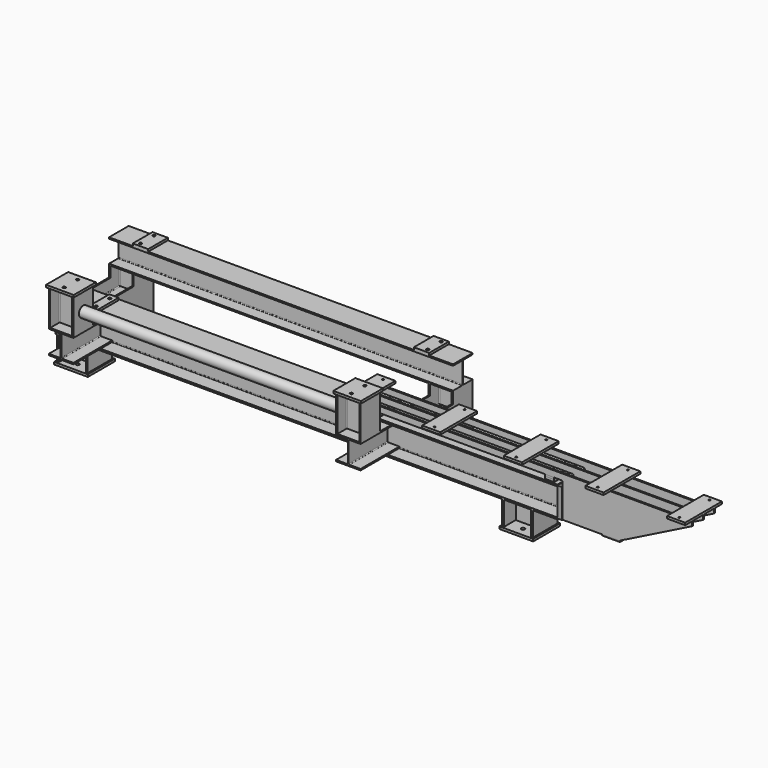
from build123d import *

# Parameters (mm, degrees)
F0_W       = 228.6
F0_H       = 228.6
F0_R       = 14.2875
F1_DEPTH   = 19.05
F0_W_2     = 279.4
F0_H_2     = 279.4
F3_DEPTH   = 504.952
F5_DEPTH   = 2844.8
F6_W       = 127
F6_H       = 203.2
F6_R       = 11.1125
F7_DEPTH   = 19.05
F9_DEPTH   = 482.6
F12_DEPTH  = 4152.9
F14_DEPTH  = 198.374
F15_W      = 76.2
F15_H      = 228.6
F15_R      = 11.1125
F16_DEPTH  = 19.05
F18_DEPTH  = 401.574
F20_DEPTH  = 292.1
F21_W      = 228.6
F21_H      = 228.6
F21_R      = 11.1125
F22_DEPTH  = 19.05
F23_R      = 44.45
F23_R_2    = 38.9636
F24_DEPTH  = 2171.7
F25_W      = 76.2
F25_H      = 228.6
F25_R      = 11.1125
F26_DEPTH  = 19
F28_W      = 150
F28_H      = 380
F28_R      = 7.25
F29_DEPTH  = 19
F31_W      = 254
F31_H      = 239.776
F31_R      = 10
F32_DEPTH  = 19
F33_W      = 254
F33_H      = 239.776
F33_R      = 10
F34_DEPTH  = 19
F36_DEPTH  = 6.25
F38_DEPTH  = 6.25
F39_SIZE2  = 600
F39_SIZE   = 300
F41_SIZE   = 40
F41_2_SIZE = 40
F43_W      = 150
F43_H      = 228.6
F44_DEPTH  = 12.5


with BuildPart() as f1:
    # F0 (on Top) → F1 (new body)
    with BuildSketch(Plane.XY):
        with Locations((-1320.8, 241.3)):
            Rectangle(F0_W, F0_H)
        with Locations((-1320.8, 171.45)):
            Circle(F0_R, mode=Mode.SUBTRACT)
        with Locations((-1320.8, 311.15)):
            Circle(F0_R, mode=Mode.SUBTRACT)
    extrude(amount=F1_DEPTH)

    # F2 (on face) → F3 (join)
    with BuildSketch(Plane.XY.offset(19.05)):
        with BuildLine():
            Line((-1411.351, 342.9), (-1422.4, 342.9))
            Line((-1422.4, 342.9), (-1422.4, 139.7))
            Line((-1422.4, 139.7), (-1411.351, 139.7))
            Line((-1411.351, 139.7), (-1411.351, 231.3305))
            ThreePointArc((-1411.351, 231.3305), (-1409.4911280605, 235.8206280605), (-1405.001, 237.6805))
            Line((-1405.001, 237.6805), (-1320.8, 237.6805))
            Line((-1320.8, 237.6805), (-1236.599, 237.6805))
            ThreePointArc((-1236.599, 237.6805), (-1232.1088719395, 235.8206280605), (-1230.249, 231.3305))
            Line((-1230.249, 231.3305), (-1230.249, 139.7))
            Line((-1230.249, 139.7), (-1219.2, 139.7))
            Line((-1219.2, 139.7), (-1219.2, 342.9))
            Line((-1219.2, 342.9), (-1230.249, 342.9))
            Line((-1230.249, 342.9), (-1230.249, 251.2695))
            ThreePointArc((-1230.249, 251.2695), (-1232.1088719395, 246.7793719395), (-1236.599, 244.9195))
            Line((-1236.599, 244.9195), (-1320.8, 244.9195))
            Line((-1320.8, 244.9195), (-1405.001, 244.9195))
            ThreePointArc((-1405.001, 244.9195), (-1409.4911280605, 246.7793719395), (-1411.351, 251.2695))
            Line((-1411.351, 251.2695), (-1411.351, 342.9))
        make_face()
    extrude(amount=F3_DEPTH)



with BuildPart() as f1b:
    # F0 (on Top) → F1, piece 2 (new body)
    with BuildSketch(Plane.XY):
        with Locations((1320.8, 241.3)):
            Rectangle(F0_W, F0_H)
        with Locations((1320.8, 171.45)):
            Circle(F0_R, mode=Mode.SUBTRACT)
        with Locations((1320.8, 311.15)):
            Circle(F0_R, mode=Mode.SUBTRACT)
    extrude(amount=F1_DEPTH)

    # F2 (on face) → F3, piece 2 (join)
    with BuildSketch(Plane.XY.offset(19.05)):
        with BuildLine():
            Line((1411.351, 342.9), (1411.351, 251.2695))
            ThreePointArc((1411.351, 251.2695), (1409.4911280605, 246.7793719395), (1405.001, 244.9195))
            Line((1405.001, 244.9195), (1320.8, 244.9195))
            Line((1320.8, 244.9195), (1236.599, 244.9195))
            ThreePointArc((1236.599, 244.9195), (1232.1088719395, 246.7793719395), (1230.249, 251.2695))
            Line((1230.249, 251.2695), (1230.249, 342.9))
            Line((1230.249, 342.9), (1219.2, 342.9))
            Line((1219.2, 342.9), (1219.2, 139.7))
            Line((1219.2, 139.7), (1230.249, 139.7))
            Line((1230.249, 139.7), (1230.249, 231.3305))
            ThreePointArc((1230.249, 231.3305), (1232.1088719395, 235.8206280605), (1236.599, 237.6805))
            Line((1236.599, 237.6805), (1320.8, 237.6805))
            Line((1320.8, 237.6805), (1405.001, 237.6805))
            ThreePointArc((1405.001, 237.6805), (1409.4911280605, 235.8206280605), (1411.351, 231.3305))
            Line((1411.351, 231.3305), (1411.351, 139.7))
            Line((1411.351, 139.7), (1422.4, 139.7))
            Line((1422.4, 139.7), (1422.4, 342.9))
            Line((1422.4, 342.9), (1411.351, 342.9))
        make_face()
    extrude(amount=F3_DEPTH)


with BuildPart() as f1c:
    # F0 (on Top) → F1, piece 3 (new body)
    with BuildSketch(Plane.XY):
        with Locations((2362.2, -241.3)):
            Rectangle(F0_W_2, F0_H_2)
        with Locations((2362.2, -311.15)):
            Circle(F0_R, mode=Mode.SUBTRACT)
        with Locations((2362.2, -171.45)):
            Circle(F0_R, mode=Mode.SUBTRACT)
    extrude(amount=F1_DEPTH)


with BuildPart() as f1d:
    # F0 (on Top) → F1, piece 4 (new body)
    with BuildSketch(Plane.XY):
        with Locations((-1320.8, -241.3)):
            Rectangle(F0_W_2, F0_H_2)
        with Locations((-1320.8, -311.15)):
            Circle(F0_R, mode=Mode.SUBTRACT)
        with Locations((-1320.8, -171.45)):
            Circle(F0_R, mode=Mode.SUBTRACT)
    extrude(amount=F1_DEPTH)


with BuildPart() as f1_1:
    add(f1.part)

    add(f1b.part)  # F5 merges F1b
    # F4 (on face) → F5 (join, through all)
    with BuildSketch(Plane.YZ.offset(1422.4)):
        with BuildLine():
            Line((139.7, 535.051), (139.7, 524.002))
            Line((139.7, 524.002), (342.9, 524.002))
            Line((342.9, 524.002), (342.9, 535.051))
            Line((342.9, 535.051), (251.2695, 535.051))
            ThreePointArc((251.2695, 535.051), (246.7793719395, 536.9108719395), (244.9195, 541.401))
            Line((244.9195, 541.401), (244.9195, 709.803))
            ThreePointArc((244.9195, 709.803), (246.7793719395, 714.2931280605), (251.2695, 716.153))
            Line((251.2695, 716.153), (342.9, 716.153))
            Line((342.9, 716.153), (342.9, 727.202))
            Line((342.9, 727.202), (139.7, 727.202))
            Line((139.7, 727.202), (139.7, 716.153))
            Line((139.7, 716.153), (231.3305, 716.153))
            ThreePointArc((231.3305, 716.153), (235.8206280605, 714.2931280605), (237.6805, 709.803))
            Line((237.6805, 709.803), (237.6805, 541.401))
            ThreePointArc((237.6805, 541.401), (235.8206280605, 536.9108719395), (231.3305, 535.051))
            Line((231.3305, 535.051), (139.7, 535.051))
        make_face()
    extrude(amount=-F5_DEPTH)

    # F6 (on face) → F7 (join)
    with BuildSketch(Plane.XY.offset(727.202)):
        with Locations((1162.05, 241.3)):
            Rectangle(F6_W, F6_H)
        with Locations((1187.45, 171.45)):
            Circle(F6_R, mode=Mode.SUBTRACT)
        with Locations((1187.45, 311.15)):
            Circle(F6_R, mode=Mode.SUBTRACT)
        with Locations((-1162.05, 241.3)):
            Rectangle(F6_W, F6_H)
        with Locations((-1187.45, 171.45)):
            Circle(F6_R, mode=Mode.SUBTRACT)
        with Locations((-1187.45, 311.15)):
            Circle(F6_R, mode=Mode.SUBTRACT)
    extrude(amount=F7_DEPTH)

    # F8 (on face) → F9 (join)
    with BuildSketch(Plane.XZ.offset(-237.6805)):
        with BuildLine():
            Line((-1422.4, 434.848), (-1422.4, 231.648))
            Line((-1422.4, 231.648), (-1411.351, 231.648))
            Line((-1411.351, 231.648), (-1411.351, 328.803))
            ThreePointArc((-1411.351, 328.803), (-1410.9790256121, 329.7010256121), (-1410.081, 330.073))
            Line((-1410.081, 330.073), (-1320.8, 330.073))
            Line((-1320.8, 330.073), (-1231.519, 330.073))
            ThreePointArc((-1231.519, 330.073), (-1230.6209743879, 329.7010256121), (-1230.249, 328.803))
            Line((-1230.249, 328.803), (-1230.249, 231.648))
            Line((-1230.249, 231.648), (-1219.2, 231.648))
            Line((-1219.2, 231.648), (-1219.2, 434.848))
            Line((-1219.2, 434.848), (-1230.249, 434.848))
            Line((-1230.249, 434.848), (-1230.249, 342.773))
            ThreePointArc((-1230.249, 342.773), (-1232.1088719395, 338.2828719395), (-1236.599, 336.423))
            Line((-1236.599, 336.423), (-1320.8, 336.423))
            Line((-1320.8, 336.423), (-1405.001, 336.423))
            ThreePointArc((-1405.001, 336.423), (-1409.4911280605, 338.2828719395), (-1411.351, 342.773))
            Line((-1411.351, 342.773), (-1411.351, 434.848))
            Line((-1411.351, 434.848), (-1422.4, 434.848))
        make_face()
        with BuildLine():
            Line((1411.351, 434.848), (1411.351, 342.773))
            ThreePointArc((1411.351, 342.773), (1409.4911280605, 338.2828719395), (1405.001, 336.423))
            Line((1405.001, 336.423), (1320.8, 336.423))
            Line((1320.8, 336.423), (1236.599, 336.423))
            ThreePointArc((1236.599, 336.423), (1232.1088719395, 338.2828719395), (1230.249, 342.773))
            Line((1230.249, 342.773), (1230.249, 434.848))
            Line((1230.249, 434.848), (1219.2, 434.848))
            Line((1219.2, 434.848), (1219.2, 231.648))
            Line((1219.2, 231.648), (1230.249, 231.648))
            Line((1230.249, 231.648), (1230.249, 328.803))
            ThreePointArc((1230.249, 328.803), (1230.6209743879, 329.7010256121), (1231.519, 330.073))
            Line((1231.519, 330.073), (1320.8, 330.073))
            Line((1320.8, 330.073), (1410.081, 330.073))
            ThreePointArc((1410.081, 330.073), (1410.9790256121, 329.7010256121), (1411.351, 328.803))
            Line((1411.351, 328.803), (1411.351, 231.648))
            Line((1411.351, 231.648), (1422.4, 231.648))
            Line((1422.4, 231.648), (1422.4, 434.848))
            Line((1422.4, 434.848), (1411.351, 434.848))
        make_face()
    extrude(amount=F9_DEPTH)

    # F11 (on offset) → F12 (join)
    with BuildSketch(Plane.YZ.offset(2692.4)):
        with BuildLine():
            Line((-368.3, 231.648), (-368.3, 217.424))
            Line((-368.3, 217.424), (-114.3, 217.424))
            Line((-114.3, 217.424), (-114.3, 231.648))
            Line((-114.3, 231.648), (-228.6, 231.648))
            ThreePointArc((-228.6, 231.648), (-233.0901280605, 233.5078719395), (-234.95, 237.998))
            Line((-234.95, 237.998), (-234.95, 450.85))
            ThreePointArc((-234.95, 450.85), (-233.0901280605, 455.3401280605), (-228.6, 457.2))
            Line((-228.6, 457.2), (-114.3, 457.2))
            Line((-114.3, 457.2), (-114.3, 471.424))
            Line((-114.3, 471.424), (-368.3, 471.424))
            Line((-368.3, 471.424), (-368.3, 457.2))
            Line((-368.3, 457.2), (-254, 457.2))
            ThreePointArc((-254, 457.2), (-249.5098719395, 455.3401280605), (-247.65, 450.85))
            Line((-247.65, 450.85), (-247.65, 237.998))
            ThreePointArc((-247.65, 237.998), (-249.5098719395, 233.5078719395), (-254, 231.648))
            Line((-254, 231.648), (-368.3, 231.648))
        make_face()
    extrude(amount=-F12_DEPTH)


    add(f1c.part)  # F14 merges F1c

    add(f1d.part)  # F14 merges F1d
    # F13 (on face) → F14 (join)
    with BuildSketch(Plane.XY.offset(19.05)):
        Polygon((-1433.576, -114.3), (-1447.8, -114.3), (-1447.8, -368.3), (-1433.576, -368.3), (-1433.576, -245.618), (-1208.024, -245.618), (-1208.024, -368.3), (-1193.8, -368.3), (-1193.8, -114.3), (-1208.024, -114.3), (-1208.024, -236.982), (-1433.576, -236.982), align=None)
        Polygon((2474.976, -368.3), (2489.2, -368.3), (2489.2, -114.3), (2474.976, -114.3), (2474.976, -236.982), (2249.424, -236.982), (2249.424, -114.3), (2235.2, -114.3), (2235.2, -368.3), (2249.424, -368.3), (2249.424, -245.618), (2474.976, -245.618), align=None)
    extrude(amount=F14_DEPTH)

    # F15 (on face) → F16 (join)
    with BuildSketch(Plane.XY.offset(471.424)):
        with Locations((-1168.4, -241.3)):
            Rectangle(F15_W, F15_H)
        with Locations((-1168.4, -311.15)):
            Circle(F15_R, mode=Mode.SUBTRACT)
        with Locations((-1168.4, -171.45)):
            Circle(F15_R, mode=Mode.SUBTRACT)
        with Locations((1168.4, -241.3)):
            Rectangle(F15_W, F15_H)
        with Locations((1168.4, -311.15)):
            Circle(F15_R, mode=Mode.SUBTRACT)
        with Locations((1168.4, -171.45)):
            Circle(F15_R, mode=Mode.SUBTRACT)
        with Locations((2616.2, -241.3)):
            Rectangle(F15_W, F15_H)
        with Locations((2616.2, -311.15)):
            Circle(F15_R, mode=Mode.SUBTRACT)
        with Locations((2616.2, -171.45)):
            Circle(F15_R, mode=Mode.SUBTRACT)
    extrude(amount=F16_DEPTH)

    # F17 (on face) → F18 (join)
    with BuildSketch(Plane.XZ.offset(247.65)):
        with BuildLine():
            Line((-1085.85, 435.102), (-1289.05, 435.102))
            Line((-1289.05, 435.102), (-1289.05, 424.053))
            Line((-1289.05, 424.053), (-1197.356, 424.053))
            ThreePointArc((-1197.356, 424.053), (-1192.8658719395, 422.1931280605), (-1191.006, 417.703))
            Line((-1191.006, 417.703), (-1191.006, 249.301))
            ThreePointArc((-1191.006, 249.301), (-1192.8658719395, 244.8108719395), (-1197.356, 242.951))
            Line((-1197.356, 242.951), (-1289.05, 242.951))
            Line((-1289.05, 242.951), (-1289.05, 231.902))
            Line((-1289.05, 231.902), (-1085.85, 231.902))
            Line((-1085.85, 231.902), (-1085.85, 242.951))
            Line((-1085.85, 242.951), (-1177.544, 242.951))
            ThreePointArc((-1177.544, 242.951), (-1182.0341280605, 244.8108719395), (-1183.894, 249.301))
            Line((-1183.894, 249.301), (-1183.894, 417.703))
            ThreePointArc((-1183.894, 417.703), (-1182.0341280605, 422.1931280605), (-1177.544, 424.053))
            Line((-1177.544, 424.053), (-1085.85, 424.053))
            Line((-1085.85, 424.053), (-1085.85, 435.102))
        make_face()
        with BuildLine():
            Line((1085.85, 424.053), (1177.544, 424.053))
            ThreePointArc((1177.544, 424.053), (1182.0341280605, 422.1931280605), (1183.894, 417.703))
            Line((1183.894, 417.703), (1183.894, 249.301))
            ThreePointArc((1183.894, 249.301), (1182.0341280605, 244.8108719395), (1177.544, 242.951))
            Line((1177.544, 242.951), (1085.85, 242.951))
            Line((1085.85, 242.951), (1085.85, 231.902))
            Line((1085.85, 231.902), (1289.05, 231.902))
            Line((1289.05, 231.902), (1289.05, 242.951))
            Line((1289.05, 242.951), (1197.356, 242.951))
            ThreePointArc((1197.356, 242.951), (1192.8658719395, 244.8108719395), (1191.006, 249.301))
            Line((1191.006, 249.301), (1191.006, 417.703))
            ThreePointArc((1191.006, 417.703), (1192.8658719395, 422.1931280605), (1197.356, 424.053))
            Line((1197.356, 424.053), (1289.05, 424.053))
            Line((1289.05, 424.053), (1289.05, 435.102))
            Line((1289.05, 435.102), (1085.85, 435.102))
            Line((1085.85, 435.102), (1085.85, 424.053))
        make_face()
    extrude(amount=F18_DEPTH)

    # F19 (on face) → F20 (join)
    with BuildSketch(Plane.XY.offset(435.102)):
        with BuildLine():
            Line((-1289.05, -446.024), (-1289.05, -649.224))
            Line((-1289.05, -649.224), (-1278.001, -649.224))
            Line((-1278.001, -649.224), (-1278.001, -557.53))
            ThreePointArc((-1278.001, -557.53), (-1276.1411280605, -553.0398719395), (-1271.651, -551.18))
            Line((-1271.651, -551.18), (-1103.249, -551.18))
            ThreePointArc((-1103.249, -551.18), (-1098.7588719395, -553.0398719395), (-1096.899, -557.53))
            Line((-1096.899, -557.53), (-1096.899, -649.224))
            Line((-1096.899, -649.224), (-1085.85, -649.224))
            Line((-1085.85, -649.224), (-1085.85, -446.024))
            Line((-1085.85, -446.024), (-1096.899, -446.024))
            Line((-1096.899, -446.024), (-1096.899, -537.718))
            ThreePointArc((-1096.899, -537.718), (-1098.7588719395, -542.2081280605), (-1103.249, -544.068))
            Line((-1103.249, -544.068), (-1271.651, -544.068))
            ThreePointArc((-1271.651, -544.068), (-1276.1411280605, -542.2081280605), (-1278.001, -537.718))
            Line((-1278.001, -537.718), (-1278.001, -446.024))
            Line((-1278.001, -446.024), (-1289.05, -446.024))
        make_face()
        with BuildLine():
            Line((1103.249, -551.18), (1271.651, -551.18))
            ThreePointArc((1271.651, -551.18), (1276.1411280605, -553.0398719395), (1278.001, -557.53))
            Line((1278.001, -557.53), (1278.001, -649.224))
            Line((1278.001, -649.224), (1289.05, -649.224))
            Line((1289.05, -649.224), (1289.05, -446.024))
            Line((1289.05, -446.024), (1278.001, -446.024))
            Line((1278.001, -446.024), (1278.001, -537.718))
            ThreePointArc((1278.001, -537.718), (1276.1411280605, -542.2081280605), (1271.651, -544.068))
            Line((1271.651, -544.068), (1103.249, -544.068))
            ThreePointArc((1103.249, -544.068), (1098.7588719395, -542.2081280605), (1096.899, -537.718))
            Line((1096.899, -537.718), (1096.899, -446.024))
            Line((1096.899, -446.024), (1085.85, -446.024))
            Line((1085.85, -446.024), (1085.85, -649.224))
            Line((1085.85, -649.224), (1096.899, -649.224))
            Line((1096.899, -649.224), (1096.899, -557.53))
            ThreePointArc((1096.899, -557.53), (1098.7588719395, -553.0398719395), (1103.249, -551.18))
        make_face()
    extrude(amount=F20_DEPTH)

    # F21 (on face) → F22 (join)
    with BuildSketch(Plane.XY.offset(727.202)):
        with Locations((-1187.45, -547.624)):
            Rectangle(F21_W, F21_H)
        with Locations((-1187.45, -617.474)):
            Circle(F21_R, mode=Mode.SUBTRACT)
        with Locations((-1187.45, -477.774)):
            Circle(F21_R, mode=Mode.SUBTRACT)
        with Locations((1187.45, -547.624)):
            Rectangle(F21_W, F21_H)
        with Locations((1187.45, -617.474)):
            Circle(F21_R, mode=Mode.SUBTRACT)
        with Locations((1187.45, -477.774)):
            Circle(F21_R, mode=Mode.SUBTRACT)
    extrude(amount=F22_DEPTH)

    # F23 (on face) → F24 (join)
    with BuildSketch(Plane.YZ.offset(-1085.85)):
        with Locations((-547.624, 574.802)):
            Circle(F23_R)
        with Locations((-547.624, 574.802)):
            Circle(F23_R_2, mode=Mode.SUBTRACT)
    extrude(amount=F24_DEPTH)


with BuildPart() as f26:
    # F25 (on face) → F26 (new body)
    with BuildSketch(Plane.XY.offset(490.474)):
        with Locations((1168.4, -241.3)):
            Rectangle(F25_W, F25_H)
        with Locations((1168.4, -311.15)):
            Circle(F25_R, mode=Mode.SUBTRACT)
        with Locations((1168.4, -171.45)):
            Circle(F25_R, mode=Mode.SUBTRACT)
    extrude(amount=F26_DEPTH)



with BuildPart() as f26b:
    # F25 (on face) → F26, piece 2 (new body)
    with BuildSketch(Plane.XY.offset(490.474)):
        with Locations((2616.2, -241.3)):
            Rectangle(F25_W, F25_H)
        with Locations((2616.2, -311.15)):
            Circle(F25_R, mode=Mode.SUBTRACT)
        with Locations((2616.2, -171.45)):
            Circle(F25_R, mode=Mode.SUBTRACT)
    extrude(amount=F26_DEPTH)


with BuildPart() as f29:
    # F28 (on offset) → F29 (new body)
    with BuildSketch(Plane.XY.offset(579.424)):
        with Locations((1023.9, -241.3)):
            Rectangle(F28_W, F28_H)
        with Locations((1023.9, -396.3)):
            Circle(F28_R, mode=Mode.SUBTRACT)
        with Locations((1023.9, -86.3)):
            Circle(F28_R, mode=Mode.SUBTRACT)
    extrude(amount=-F29_DEPTH)


with BuildPart() as f29b:
    # F28 (on offset) → F29, piece 2 (new body)
    with BuildSketch(Plane.XY.offset(579.424)):
        with Locations((1698.9, -241.3)):
            Rectangle(F28_W, F28_H)
        with Locations((1698.9, -396.3)):
            Circle(F28_R, mode=Mode.SUBTRACT)
        with Locations((1698.9, -86.3)):
            Circle(F28_R, mode=Mode.SUBTRACT)
    extrude(amount=-F29_DEPTH)


with BuildPart() as f29c:
    # F28 (on offset) → F29, piece 3 (new body)
    with BuildSketch(Plane.XY.offset(579.424)):
        with Locations((2373.9, -241.3)):
            Rectangle(F28_W, F28_H)
        with Locations((2373.9, -396.3)):
            Circle(F28_R, mode=Mode.SUBTRACT)
        with Locations((2373.9, -86.3)):
            Circle(F28_R, mode=Mode.SUBTRACT)
    extrude(amount=-F29_DEPTH)


with BuildPart() as f29d:
    # F28 (on offset) → F29, piece 4 (new body)
    with BuildSketch(Plane.XY.offset(579.424)):
        with Locations((3048.9, -241.3)):
            Rectangle(F28_W, F28_H)
        with Locations((3048.9, -396.3)):
            Circle(F28_R, mode=Mode.SUBTRACT)
        with Locations((3048.9, -86.3)):
            Circle(F28_R, mode=Mode.SUBTRACT)
    extrude(amount=-F29_DEPTH)


with BuildPart() as f29e:
    # F28 (on offset) → F29, piece 5 (new body)
    with BuildSketch(Plane.XY.offset(579.424)):
        with Locations((3723.9, -241.3)):
            Rectangle(F28_W, F28_H)
        with Locations((3723.9, -396.3)):
            Circle(F28_R, mode=Mode.SUBTRACT)
        with Locations((3723.9, -86.3)):
            Circle(F28_R, mode=Mode.SUBTRACT)
    extrude(amount=-F29_DEPTH)


with BuildPart() as f32:
    # F31 (on offset) → F32 (new body)
    with BuildSketch(Plane.YZ.offset(2692.4)):
        with Locations((-241.3, 344.424)):
            Rectangle(F31_W, F31_H)
        with Locations((-318.3, 264.424)):
            Circle(F31_R, mode=Mode.SUBTRACT)
        with Locations((-318.3, 344.424)):
            Circle(F31_R, mode=Mode.SUBTRACT)
        with Locations((-164.3, 264.424)):
            Circle(F31_R, mode=Mode.SUBTRACT)
        with Locations((-164.3, 344.424)):
            Circle(F31_R, mode=Mode.SUBTRACT)
        with Locations((-318.3, 424.424)):
            Circle(F31_R, mode=Mode.SUBTRACT)
        with Locations((-164.3, 424.424)):
            Circle(F31_R, mode=Mode.SUBTRACT)
    extrude(amount=F32_DEPTH)


with BuildPart() as f34:
    # F33 (on face) → F34 (new body)
    with BuildSketch(Plane.YZ.offset(2711.4)):
        with Locations((-241.3, 344.424)):
            Rectangle(F33_W, F33_H)
        with Locations((-318.3, 264.424)):
            Circle(F33_R, mode=Mode.SUBTRACT)
        with Locations((-318.3, 344.424)):
            Circle(F33_R, mode=Mode.SUBTRACT)
        with Locations((-164.3, 264.424)):
            Circle(F33_R, mode=Mode.SUBTRACT)
        with Locations((-164.3, 344.424)):
            Circle(F33_R, mode=Mode.SUBTRACT)
        with Locations((-318.3, 424.424)):
            Circle(F33_R, mode=Mode.SUBTRACT)
        with Locations((-164.3, 424.424)):
            Circle(F33_R, mode=Mode.SUBTRACT)
    extrude(amount=F34_DEPTH)


with BuildPart() as f26_1:
    add(f26.part)

    add(f26b.part)  # F36 merges F26b

    add(f29.part)  # F36 merges F29

    add(f29b.part)  # F36 merges F29b

    add(f29c.part)  # F36 merges F29c

    add(f29d.part)  # F36 merges F29d

    add(f29e.part)  # F36 merges F29e

    add(f34.part)  # F36 merges F34
    # F35 (on mid) → F36 (join, symmetric)
    with BuildSketch(Plane.XZ.offset(241.3)):
        with BuildLine():
            Line((3798.9, 560.424), (948.9, 560.424))
            Line((948.9, 560.424), (948.9, 509.474))
            Line((948.9, 509.474), (2720.4, 509.474))
            ThreePointArc((2720.4, 509.474), (2727.4710678119, 506.5450678119), (2730.4, 499.474))
            Line((2730.4, 499.474), (2730.4, 464.312))
            Line((2730.4, 464.312), (2730.4, 224.536))
            Line((2730.4, 224.536), (3798.9, 224.536))
            Line((3798.9, 224.536), (3798.9, 560.424))
        make_face()
    extrude(amount=F36_DEPTH, both=True)

    # F37 (on face) → F38 (join, symmetric)
    with BuildSketch(Plane.XZ.offset(355.6)):
        with BuildLine():
            Line((3798.9, 224.536), (3798.9, 560.424))
            Line((3798.9, 560.424), (948.9, 560.424))
            Line((948.9, 560.424), (948.9, 509.474))
            Line((948.9, 509.474), (2720.4, 509.474))
            ThreePointArc((2720.4, 509.474), (2727.4710678119, 506.5450678119), (2730.4, 499.474))
            Line((2730.4, 499.474), (2730.4, 224.536))
            Line((2730.4, 224.536), (3798.9, 224.536))
        make_face()
    extrude(amount=F38_DEPTH, both=True)

    # F39
    f39_edges = [f26_1.edges().sort_by_distance(p)[0] for p in [
        (3798.9, -241.3, 224.536),
        (3798.9, -355.6, 224.536),
    ]]
    f39_side = f26_1.faces().sort_by_distance((3798.9, -426.100524, 569.924))[0]
    chamfer(f39_edges, length=F39_SIZE, length2=F39_SIZE2, reference=f39_side)


with BuildPart() as f40_1:
    # F40: instance of F26
    add(f26_1.part.mirror(Plane(origin=(1168.4, -241.3, 499.974), x_dir=(1, 0, 0), z_dir=(0, -1, 0))))

    # F41#2
    f41_2_edges = [f40_1.edges().sort_by_distance(p)[0] for p in [
        (948.9, -241.3, 509.474),
        (948.9, -127, 509.474),
    ]]
    chamfer(f41_2_edges, length=F41_2_SIZE)


with BuildPart() as f26_2:
    add(f26_1.part)

    # F41
    f41_edges = [f26_2.edges().sort_by_distance(p)[0] for p in [
        (948.9, -241.3, 509.474),
        (948.9, -355.6, 509.474),
    ]]
    chamfer(f41_edges, length=F41_SIZE)

    # F42: union F40_1
    add(f40_1.part)

    # F43 (on face) → F44 (join)
    with BuildSketch(Plane(origin=(0, 0, 224.536), x_dir=(1, 0, 0), z_dir=(0, 0, -1))):
        with Locations((3123.9, 241.3)):
            Rectangle(F43_W, F43_H)
    extrude(amount=F44_DEPTH)


solid = Compound([f1_1.part, f32.part, f26_2.part])
